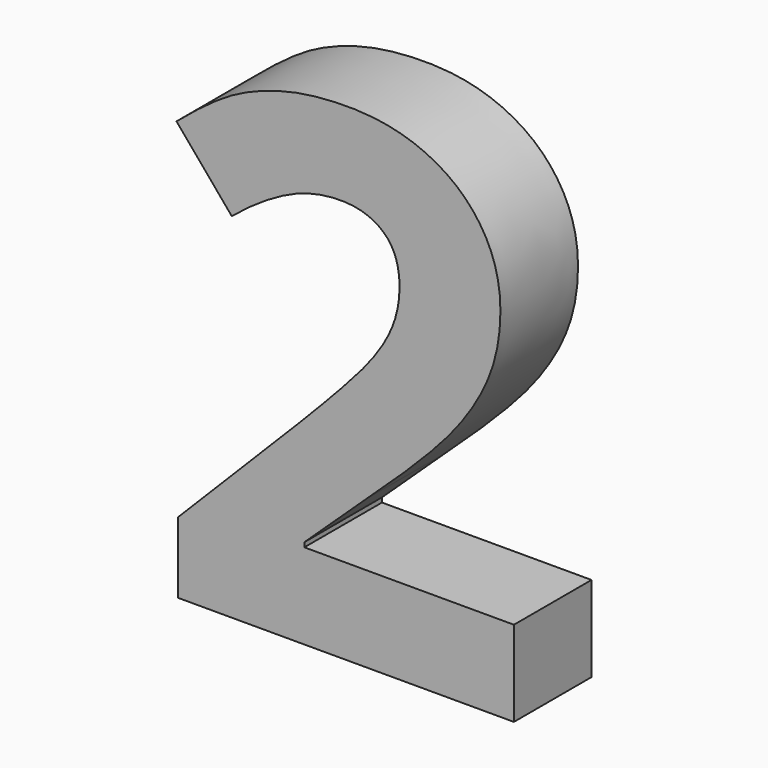
from build123d import *

# Parameters (mm, degrees)
F0_TEXT_SIZE = 35.2777777778
F1_DEPTH     = 5.08


# Not quite as in the source:
# - Text() gives the source's letters only with a copy of the font that has no kerning and outlines rounded to 1/6400 em; it was checked with that copy


with BuildPart() as f1:
    # F0 (on Front) → F1 (new body)
    with BuildSketch(Plane.XZ):
        with Locations((-21.3044704861, 37.3313542945)):
            Text('2', F0_TEXT_SIZE, font='Open Sans', font_style=FontStyle.BOLD, text_align=(TextAlign.LEFT, TextAlign.BOTTOM))
    extrude(amount=F1_DEPTH)


solid = f1.part
